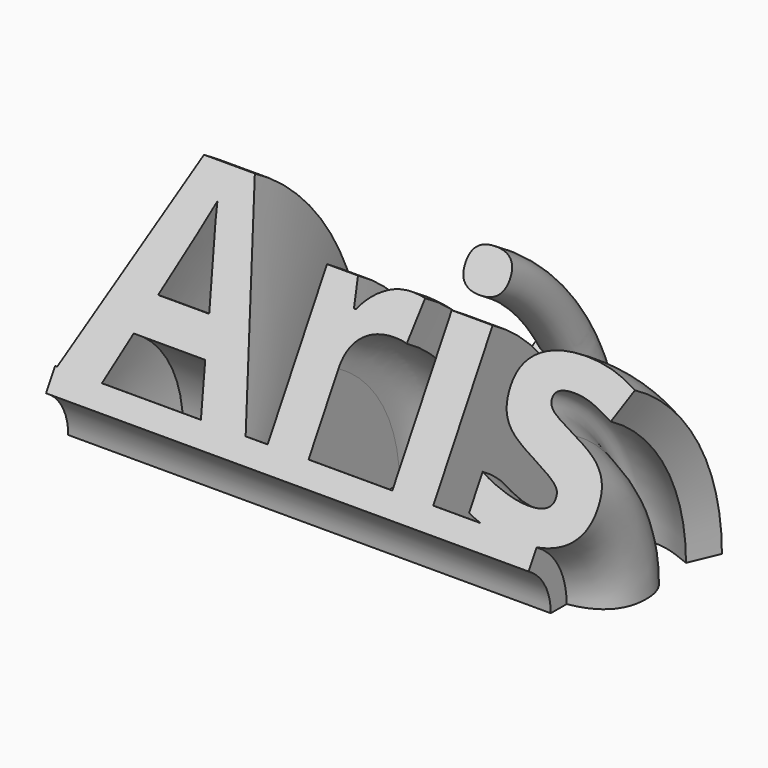
from build123d import *

# Parameters (mm, degrees)
F0_TEXT_SIZE = 49.5557440445
F1_W         = 87.0458
F1_H         = 4.0545612574
F4_ANGLE     = 60
F2_W         = 7.2898
F2_H         = 5.1357774064
F5_ANGLE     = 30


# Not quite as in the source:
# - Text() gives the source's letters only with a copy of the font that has no kerning and outlines rounded to 1/6400 em; it was checked with that copy


with BuildPart() as f4:
    # F0 (on Top) + F1 (on Top) → F4 (revolve)
    with BuildSketch(Plane.XY):
        with Locations((-76.6987800598, -18.5834039003)):
            Text('Aris', F0_TEXT_SIZE, font='Open Sans', font_style=FontStyle.BOLD, text_align=(TextAlign.LEFT, TextAlign.BOTTOM))
    with BuildSketch(Plane.XY):
        with Locations((-33.4540754853, -20.3403793275)):
            Rectangle(F1_W, F1_H)
    revolve(axis=Axis((-26.4191342531, -32.3689095676, 0), (1, 0, 0)), revolution_arc=F4_ANGLE)

    # F2 (on Top) → F5 (revolve)
    with BuildSketch(Plane.XY):
        with Locations((-12.5057682634, 11.0148903914)):
            Rectangle(F2_W, F2_H)
    revolve(axis=Axis((-26.4191342531, -32.3689095676, 0), (1, 0, 0)), revolution_arc=F5_ANGLE)


solid = f4.part
